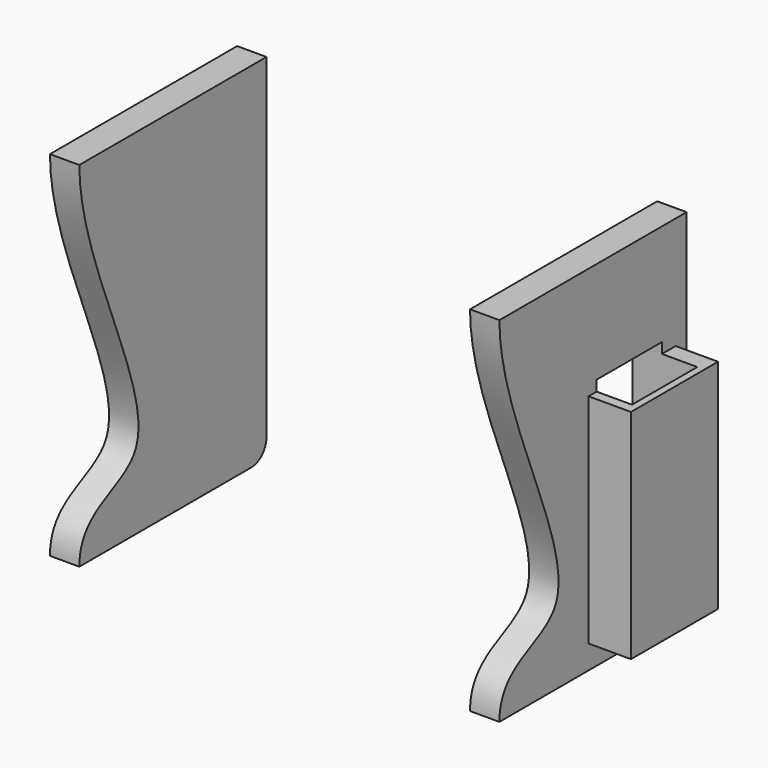
from build123d import *

# Parameters (mm, degrees)
F0_R      = 1.75
F1_DEPTH  = 3
F3_DEPTH  = 41.3
F5_DEPTH  = 5.4
F6_W      = 20
F6_H      = 40
F7_DEPTH  = 49.1
F8_DEPTH  = 25
F9_W      = 15
F9_H      = 40.159
F10_DEPTH = 47.8


# Not quite as in the source:
# - a feature names something its author has since deleted; it is built from what else it names


with BuildPart() as f1:
    # F0 (on Top) → F1 (new body)
    with BuildSketch(Plane.XY):
        with BuildLine():
            Line((-41.5, -22.5), (41.5, -22.5))
            ThreePointArc((41.5, -22.5), (43.9748737342, -21.4748737342), (45, -19))
            Line((45, -19), (45, 19))
            ThreePointArc((45, 19), (43.9748737342, 21.4748737342), (41.5, 22.5))
            Line((41.5, 22.5), (-41.5, 22.5))
            ThreePointArc((-41.5, 22.5), (-43.9748737342, 21.4748737342), (-45, 19))
            Line((-45, 19), (-45, -19))
            ThreePointArc((-45, -19), (-43.9748737342, -21.4748737342), (-41.5, -22.5))
        make_face()
        with Locations((-30, -7.5)):
            Circle(F0_R, mode=Mode.SUBTRACT)
        with Locations((-15, -7.5)):
            Circle(F0_R, mode=Mode.SUBTRACT)
        with Locations((0, -7.5)):
            Circle(F0_R, mode=Mode.SUBTRACT)
        with Locations((15, -7.5)):
            Circle(F0_R, mode=Mode.SUBTRACT)
        with Locations((30, -7.5)):
            Circle(F0_R, mode=Mode.SUBTRACT)
        with Locations((-30, 7.5)):
            Circle(F0_R, mode=Mode.SUBTRACT)
        with Locations((-15, 7.5)):
            Circle(F0_R, mode=Mode.SUBTRACT)
        with Locations((0, 7.5)):
            Circle(F0_R, mode=Mode.SUBTRACT)
        with Locations((15.1128452271, 7.5)):
            Circle(F0_R, mode=Mode.SUBTRACT)
        with Locations((30, 7.5)):
            Circle(F0_R, mode=Mode.SUBTRACT)
    extrude(amount=F1_DEPTH)

    # F2 (on Right) → F3 (join, symmetric)
    with BuildSketch(Plane.YZ):
        with BuildLine():
            Line((20.66504623, -61.5), (20.66504623, 0))
            Line((20.66504623, 0), (-22.33495377, 0))
            add(Edge.make_bspline(
                [(-22.33495377, 0), (-22.33495377, -17.2751359642), (5.181919243, -57.6798408053), (-22.33495377, -55.771779269), (-22.33495377, -65)],
                knots=[0, 0, 0, 0, 0.6264206586, 1, 1, 1, 1], degree=3))
            Line((-22.33495377, -65), (17.16504623, -65))
            ThreePointArc((17.16504623, -65), (19.6399199641, -63.9748737342), (20.66504623, -61.5))
        make_face()
    extrude(amount=F3_DEPTH, both=True)

    # F5 (intersect, symmetric): faces of the model
    f5_faces = [f1.faces().sort_by_distance(p)[0] for p in [
        (-41.3, 2.0507565741, -31.3637201266),
        (41.3, 2.0507565741, -31.3637201266),
    ]]
    extrude(f5_faces, amount=F5_DEPTH, both=True, dir=(-1, 0, 0), mode=Mode.INTERSECT)

    # F6 (on Right) → F7 (join)
    with BuildSketch(Plane.YZ):
        with Locations((8.1445764424, -40.6413669884)):
            Rectangle(F6_W, F6_H)
    extrude(amount=F7_DEPTH)

    # F8 (cut): a face of the model
    f8_faces = [f1.faces().sort_by_distance(p)[0] for p in [
        (17.95, 18.1445764424, -40.6413669884),
    ]]
    extrude(f8_faces, amount=-F8_DEPTH, mode=Mode.SUBTRACT)

    # F9 (on Right) → F10 (cut)
    with BuildSketch(Plane.YZ):
        with Locations((7.5, -38.7948798435)):
            Rectangle(F9_W, F9_H)
    extrude(amount=F10_DEPTH, mode=Mode.SUBTRACT)


solid = f1.part
